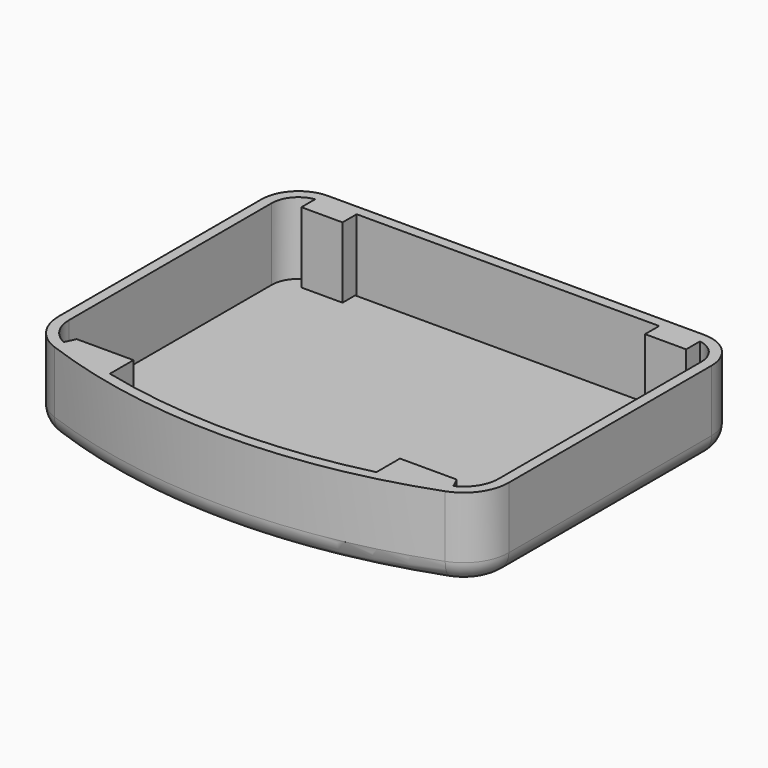
from build123d import *

# Parameters (mm, degrees)
F1_DEPTH = 25.4
F2_T     = -3.175
F3_R     = 6.35
F5_W     = 12.7
F5_H     = 6.35
F6_DEPTH = 21.844


# Not quite as in the source:
# - a feature names something its author has since deleted; it is built from what else it names


with BuildPart() as f1:
    # F0 (on Top) → F1 (new body)
    with BuildSketch(Plane.XY):
        with BuildLine():
            Line((58.0965084505, 62.5356453779), (-58.0965084505, 62.5356453779))
            ThreePointArc((-58.0965084505, 62.5356453779), (-66.1787389595, 59.1878758868), (-69.5265084505, 51.1056453779))
            Line((-69.5265084505, 51.1056453779), (-69.5265084505, -27.1992570698))
            ThreePointArc((-69.5265084505, -27.1992570698), (-67.0115325937, -35.1957139026), (-60.3721316603, -40.3130159932))
            ThreePointArc((-60.3721316603, -40.3130159932), (0, -51.0474727306), (60.3721316603, -40.3130159932))
            ThreePointArc((60.3721316603, -40.3130159932), (67.0115325937, -35.1957139026), (69.5265084505, -27.1992570698))
            Line((69.5265084505, -27.1992570698), (69.5265084505, 51.1056453779))
            ThreePointArc((69.5265084505, 51.1056453779), (66.1787389595, 59.1878758868), (58.0965084505, 62.5356453779))
        make_face()
    extrude(amount=F1_DEPTH)

    # F2
    f2_openings = [f1.faces().sort_by_distance(p)[0] for p in [
        (0, 7.919531, 25.4),
    ]]
    offset(amount=F2_T, openings=f2_openings)

    # F3
    f3_edges = [f1.edges().sort_by_distance(p)[0] for p in [
        (69.526508, 11.953194, 0),
        (66.178739, 59.187876, 0),
        (0, 62.535645, 0),
        (-66.178739, 59.187876, 0),
        (-69.526508, 11.953194, 0),
        (-67.011533, -35.195714, 0),
        (0, -51.047473, 0),
        (67.011533, -35.195714, 0),
    ]]
    fillet(f3_edges, radius=F3_R)

    # F5 (on offset) → F6 (join)
    with BuildSketch(Plane.XY.offset(25.4)):
        with Locations((-53.0805146158, 57.0815077901)):
            Rectangle(F5_W, F5_H)
        with Locations((53.0805146158, 57.0815077901)):
            Rectangle(F5_W, F5_H)
        Polygon((-41.1578565836, -33.773638308), (-58.6946308613, -33.773638308), (-60.6418885291, -37.9110425711), (-53.9016760886, -40.266495198), (-41.1578565836, -43.8219420612), align=None)
        Polygon((60.6418885291, -37.9110425711), (58.6946308613, -33.773638308), (41.1578565836, -33.773638308), (41.1578565836, -43.8219420612), (53.9016760886, -40.266495198), align=None)
    extrude(amount=-F6_DEPTH)


solid = f1.part
